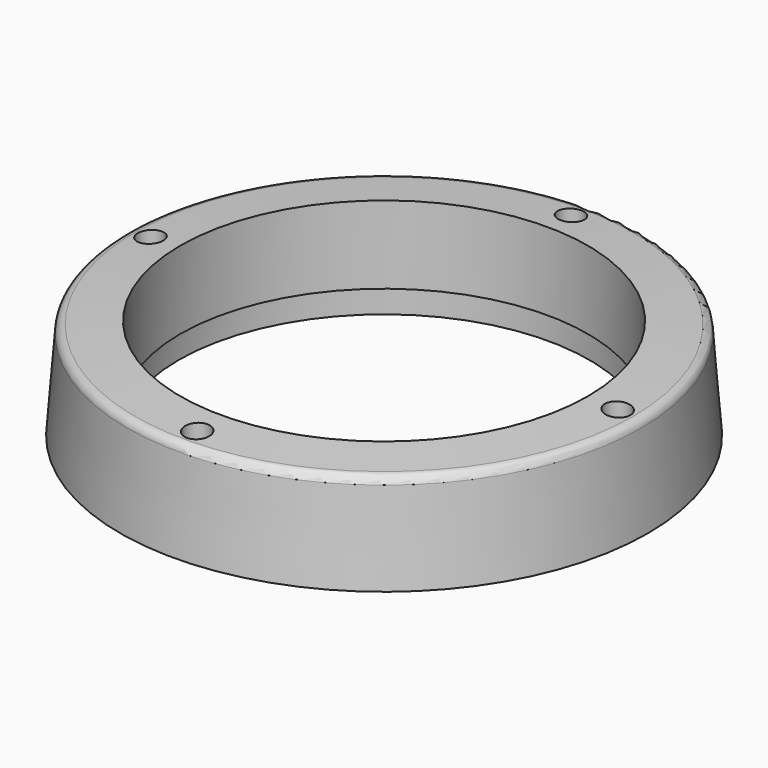
from build123d import *

# Parameters (mm, degrees)
F3_START = -14
F2_R     = 3
F3_DEPTH = 10


with BuildPart() as f1:
    # F0 (on Front) → F1 (revolve)
    with BuildSketch(Plane.XZ):
        with BuildLine():
            Line((48.35, 0), (62.15, 0))
            Line((62.15, 0), (60.5, 21.2590787789))
            ThreePointArc((60.5, 21.2590787789), (59.9118794302, 22.5268121601), (58.6373248293, 23.1))
            Line((58.6373248293, 23.1), (48, 23.8))
            Line((48, 23.8), (48, 5.5))
            Line((48, 5.5), (48.35, 5.5))
            Line((48.35, 5.5), (48.35, 0))
        make_face()
    revolve(axis=Axis((0, 0, 11.9790900654), (0, 0, 1)))

    # F2 (on face) → F3 (cut)
    with BuildSketch(Plane(origin=(0, 0, 0), x_dir=(1, 0, 0), z_dir=(0, 0, -1)).offset(F3_START)):
        with Locations((-55, 0)):
            Circle(F2_R)
        with Locations((0, 55)):
            Circle(F2_R)
        with Locations((55, 0)):
            Circle(F2_R)
        with Locations((0, -55)):
            Circle(F2_R)
    extrude(amount=-F3_DEPTH, mode=Mode.SUBTRACT)


solid = f1.part
